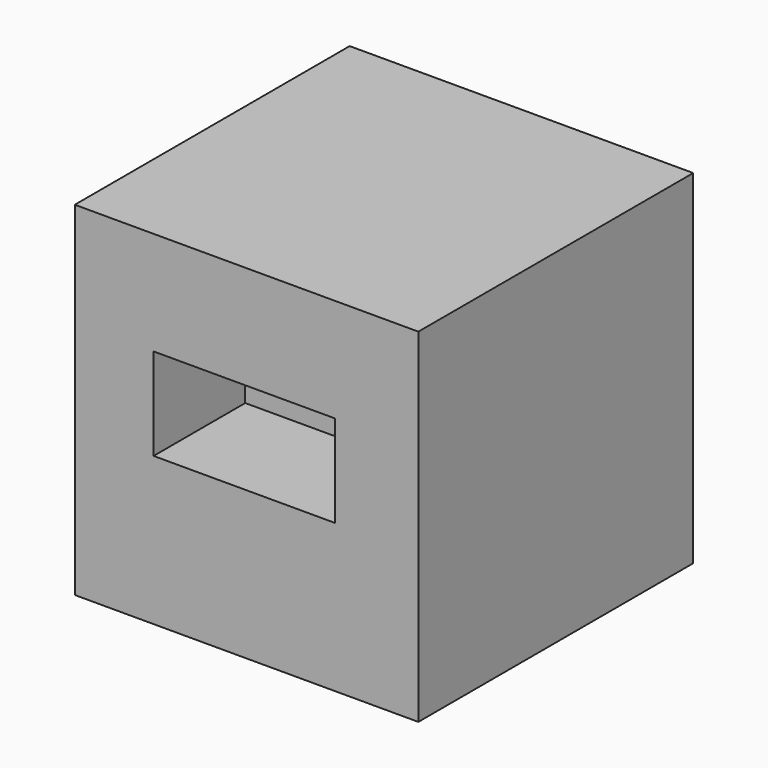
from build123d import *

# Parameters (mm, degrees)
F1_W     = 76.2
F1_H     = 76.2
F2_DEPTH = 38.1
F3_W     = 40.1978772134
F3_H     = 20.4053004272
F4_DEPTH = 25.4


# Not quite as in the source:
# - a variable given as a bare number and used for a length is read in inches; the dataset says mm whatever the document's units were


with BuildPart() as f2:
    # F1 (on Front) → F2 (new body, symmetric)
    with BuildSketch(Plane.XZ):
        Rectangle(F1_W, F1_H)
    extrude(amount=F2_DEPTH, both=True)

    # F3 (on face) → F4 (cut)
    with BuildSketch(Plane.XZ.offset(38.1)):
        with Locations((-0.5212100223, 4.9419447314)):
            Rectangle(F3_W, F3_H)
    extrude(amount=-F4_DEPTH, mode=Mode.SUBTRACT)


solid = f2.part
